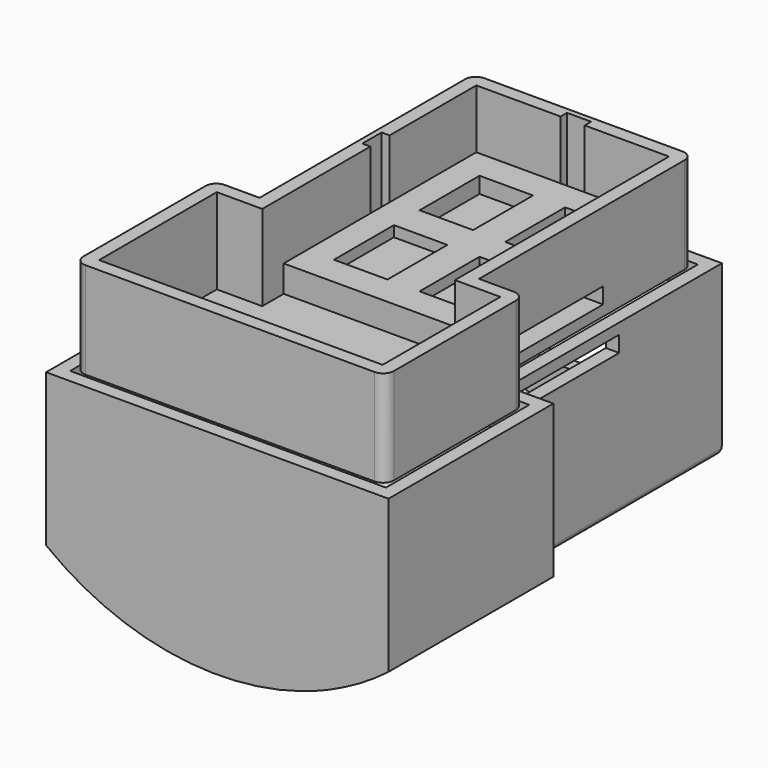
from build123d import *

# Parameters (mm, degrees)
F1_DEPTH  = 2
F2_DEPTH  = 18
F4_DEPTH  = 5
F5_W      = 24
F5_H      = 3
F6_DEPTH  = 41
F7_W      = 10
F7_H      = 14
F8_DEPTH  = 3
F9_DEPTH  = 35
F11_DEPTH = 2
F12_R     = 2
F13_W     = 31
F13_H     = 25
F14_DEPTH = 2.5
F15_R     = 10
F17_DEPTH = 50
F18_DEPTH = 50
F20_DEPTH = 38.5
F21_DEPTH = 38.5
F22_R     = 1
F23_W     = 24
F23_H     = 3
F24_DEPTH = 47
F25_SIZE2 = 20
F25_SIZE  = 2


with BuildPart() as f1:
    # F0 (on Top) → F1 (new body)
    with BuildSketch(Plane.XY):
        Polygon((20.5, -25), (20.5, 25), (-20.5, 25), (-20.5, -25), (-29, -25), (-29, -57.5), (29, -57.5), (29, -25), align=None)
        Polygon((2.25, 22.5), (18, 22.5), (18, -27.5), (26.5, -27.5), (26.5, -55), (-26.5, -55), (-26.5, -27.5), (-18, -27.5), (-18, -2.25), (-19.5, -2.25), (-19.5, 2.25), (-18, 2.25), (-18, 22.5), (-2.25, 22.5), (-2.25, 24), (2.25, 24), align=None, mode=Mode.SUBTRACT)
        Polygon((18, -27.5), (18, 22.5), (2.25, 22.5), (2.25, 24), (-2.25, 24), (-2.25, 22.5), (-18, 22.5), (-18, 2.25), (-19.5, 2.25), (-19.5, -2.25), (-18, -2.25), (-18, -27.5), (-26.5, -27.5), (-26.5, -55), (26.5, -55), (26.5, -27.5), align=None)
    extrude(amount=F1_DEPTH)

    # F0 (on Top) → F2 (join)
    with BuildSketch(Plane.XY):
        Polygon((20.5, -25), (20.5, 25), (-20.5, 25), (-20.5, -25), (-29, -25), (-29, -57.5), (29, -57.5), (29, -25), align=None)
        Polygon((2.25, 22.5), (18, 22.5), (18, -27.5), (26.5, -27.5), (26.5, -55), (-26.5, -55), (-26.5, -27.5), (-18, -27.5), (-18, -2.25), (-19.5, -2.25), (-19.5, 2.25), (-18, 2.25), (-18, 22.5), (-2.25, 22.5), (-2.25, 24), (2.25, 24), align=None, mode=Mode.SUBTRACT)
    extrude(amount=F2_DEPTH)

    # F3 (on face) → F4 (join)
    with BuildSketch(Plane.XY.offset(2)):
        Polygon((18, -22.5), (18, 22.5), (2.25, 22.5), (-2.25, 22.5), (-18, 22.5), (-18, 2.25), (-18, -2.25), (-18, -22.5), align=None)
    extrude(amount=F4_DEPTH)

    # F5 (on face) → F6 (cut, through all)
    with BuildSketch(Plane(origin=(-20.5, 0, 0), x_dir=(0, -1, 0), z_dir=(-1, 0, 0))):
        with Locations((8, 3.5)):
            Rectangle(F5_W, F5_H)
    extrude(amount=-F6_DEPTH, mode=Mode.SUBTRACT)

    # F7 (on face) → F8 (cut)
    with BuildSketch(Plane.XY.offset(7)):
        with Locations((-8, 10)):
            Rectangle(F7_W, F7_H)
        with Locations((8, 10)):
            Rectangle(F7_W, F7_H)
        with Locations((-8, -10)):
            Rectangle(F7_W, F7_H)
        with Locations((8, -10)):
            Rectangle(F7_W, F7_H)
    extrude(amount=-F8_DEPTH, mode=Mode.SUBTRACT)

    # F12
    f12_edges = [f1.edges().sort_by_distance(p)[0] for p in [
        (-29, -57.5, 9),
        (-29, -25, 9),
        (29, -57.5, 9),
        (-20.5, 25, 9),
        (29, -25, 9),
        (20.5, 25, 9),
    ]]
    fillet(f12_edges, radius=F12_R)


with BuildPart() as f9:
    # F0 (on Top) → F9 (new body)
    with BuildSketch(Plane.XY):
        Polygon((-23.5, -22), (-32, -22), (-32, -60.5), (32, -60.5), (32, -22), (23.5, -22), (23.5, 28), (-23.5, 28), align=None)
        with BuildLine():
            Line((-29.5, -58), (-29.5, -24.5))
            Line((-29.5, -24.5), (-23, -24.5))
            ThreePointArc((-23, -24.5), (-21.5857864376, -23.9142135624), (-21, -22.5))
            Line((-21, -22.5), (-21, 25.5))
            Line((-21, 25.5), (21, 25.5))
            Line((21, 25.5), (21, -22.5))
            ThreePointArc((21, -22.5), (21.5857864376, -23.9142135624), (23, -24.5))
            Line((23, -24.5), (29.5, -24.5))
            Line((29.5, -24.5), (29.5, -58))
            Line((29.5, -58), (-29.5, -58))
        make_face(mode=Mode.SUBTRACT)
    extrude(amount=-F9_DEPTH)

    # F10 (on face) → F11 (join)
    with BuildSketch(Plane(origin=(0, 0, -35), x_dir=(1, 0, 0), z_dir=(0, 0, -1))):
        Polygon((32, 60.5), (-32, 60.5), (-32, 22), (-23.5, 22), (-23.5, -28), (23.5, -28), (23.5, 22), (32, 22), align=None)
    extrude(amount=F11_DEPTH)

    # F13 (on face) → F14 (cut, through all)
    with BuildSketch(Plane(origin=(0, 28, 0), x_dir=(-1, 0, 0), z_dir=(0, 1, 0))):
        with Locations((0, -12.5)):
            Rectangle(F13_W, F13_H)
    extrude(amount=-F14_DEPTH, mode=Mode.SUBTRACT)

    # F15
    f15_edges = [f9.edges().sort_by_distance(p)[0] for p in [
        (15.5, 26.75, -25),
        (-15.5, 26.75, -25),
    ]]
    fillet(f15_edges, radius=F15_R)

    # F16 (on face) → F17 (cut, through all)
    with BuildSketch(Plane(origin=(0, 28, 0), x_dir=(-1, 0, 0), z_dir=(0, 1, 0))):
        with BuildLine():
            Line((23.5, -37), (1.547e-07, -37))
            Line((1.547e-07, -37), (-23.5, -37))
            Line((-23.5, -37), (-23.5, -37.7059200294))
            ThreePointArc((-23.5, -37.7059200294), (0, -42.9791666667), (23.5, -37.7059200294))
            Line((23.5, -37.7059200294), (23.5, -37))
        make_face()
        with BuildLine():
            ThreePointArc((1.547e-07, -37), (-12.1269327607, -35.476320292), (-23.5, -31))
            Line((-23.5, -31), (-23.5, -37))
            Line((-23.5, -37), (1.547e-07, -37))
        make_face()
        with BuildLine():
            Line((23.5, -37), (23.5, -31))
            ThreePointArc((23.5, -31), (12.1269329106, -35.4763202538), (1.547e-07, -37))
            Line((1.547e-07, -37), (23.5, -37))
        make_face()
    extrude(amount=-F17_DEPTH, mode=Mode.SUBTRACT)

    # F16 (on face) → F18 (join, through all)
    with BuildSketch(Plane(origin=(0, 28, 0), x_dir=(-1, 0, 0), z_dir=(0, 1, 0))):
        with BuildLine():
            ThreePointArc((23.5, -25), (0, -32.6310333807), (-23.5, -25))
            Line((-23.5, -25), (-23.5, -31))
            ThreePointArc((-23.5, -31), (-12.1269327607, -35.476320292), (1.547e-07, -37))
            ThreePointArc((1.547e-07, -37), (12.1269329106, -35.4763202538), (23.5, -31))
            Line((23.5, -31), (23.5, -25))
        make_face()
    extrude(amount=-F18_DEPTH)

    # F19 (on face) → F20 (cut, through all)
    with BuildSketch(Plane(origin=(0, -22, 0), x_dir=(-1, 0, 0), z_dir=(0, 1, 0))):
        with BuildLine():
            ThreePointArc((-21, -34.9837240518), (-26.6983501126, -32.0711934239), (-32, -28.4869867981))
            Line((-32, -28.4869867981), (-32, -37))
            Line((-32, -37), (-15.5852542827, -37))
            ThreePointArc((-15.5852542827, -37), (-18.3013018384, -36.073511616), (-20.962667627, -35))
            Line((-20.962667627, -35), (-21, -35))
            Line((-21, -35), (-21, -34.9837240518))
        make_face()
        with BuildLine():
            Line((-15.5852542827, -37), (-32, -37))
            Line((-32, -37), (-32, -37.6209894166))
            ThreePointArc((-32, -37.6209894166), (0, -46.8666792548), (32, -37.6209894166))
            Line((32, -37.6209894166), (32, -28.4869867981))
            ThreePointArc((32, -28.4869867981), (9.2454755251, -38.5461837253), (-15.5852542827, -37))
        make_face()
        with BuildLine():
            ThreePointArc((-23.5, -31), (-27.8967129385, -28.3609367759), (-32, -25.2854246794))
            Line((-32, -25.2854246794), (-32, -28.4869867981))
            ThreePointArc((-32, -28.4869867981), (-26.6983501126, -32.0711934239), (-21, -34.9837240518))
            Line((-21, -34.9837240518), (-21, -32.2741110813))
            ThreePointArc((-21, -32.2741110813), (-22.2591181263, -31.6549466933), (-23.5, -31))
        make_face()
        with BuildLine():
            ThreePointArc((32, -25.2854246794), (5.1211905621, -36.6037218611), (-23.5, -31))
            ThreePointArc((-23.5, -31), (-22.2591181263, -31.6549466933), (-21, -32.2741110813))
            Line((-21, -32.2741110813), (-21, -34.9837240518))
            ThreePointArc((-21, -34.9837240518), (-20.9813353917, -34.9918656459), (-20.962667627, -35))
            Line((-20.962667627, -35), (-13.859413167, -35))
            ThreePointArc((-13.859413167, -35), (-7.0014879371, -36.4974237186), (0, -37))
            Line((0, -37), (-15.5852542827, -37))
            ThreePointArc((-15.5852542827, -37), (9.2454755251, -38.5461837253), (32, -28.4869867981))
            Line((32, -28.4869867981), (32, -25.2854246794))
        make_face()
    extrude(amount=-F20_DEPTH, mode=Mode.SUBTRACT)

    # F19 (on face) → F21 (join, through all)
    with BuildSketch(Plane(origin=(0, -22, 0), x_dir=(-1, 0, 0), z_dir=(0, 1, 0))):
        with BuildLine():
            ThreePointArc((-23.5, -31), (-27.8967129385, -28.3609367759), (-32, -25.2854246794))
            Line((-32, -25.2854246794), (-32, -28.4869867981))
            ThreePointArc((-32, -28.4869867981), (-26.6983501126, -32.0711934239), (-21, -34.9837240518))
            Line((-21, -34.9837240518), (-21, -32.2741110813))
            ThreePointArc((-21, -32.2741110813), (-22.2591181263, -31.6549466933), (-23.5, -31))
        make_face()
        with BuildLine():
            Line((-13.859413167, -35), (-20.962667627, -35))
            ThreePointArc((-20.962667627, -35), (-18.3013018384, -36.073511616), (-15.5852542827, -37))
            Line((-15.5852542827, -37), (0, -37))
            ThreePointArc((0, -37), (-7.0014879371, -36.4974237186), (-13.859413167, -35))
        make_face()
        with BuildLine():
            ThreePointArc((32, -25.2854246794), (5.1211905621, -36.6037218611), (-23.5, -31))
            ThreePointArc((-23.5, -31), (-22.2591181263, -31.6549466933), (-21, -32.2741110813))
            Line((-21, -32.2741110813), (-21, -34.9837240518))
            ThreePointArc((-21, -34.9837240518), (-20.9813353917, -34.9918656459), (-20.962667627, -35))
            Line((-20.962667627, -35), (-13.859413167, -35))
            ThreePointArc((-13.859413167, -35), (-7.0014879371, -36.4974237186), (0, -37))
            Line((0, -37), (-15.5852542827, -37))
            ThreePointArc((-15.5852542827, -37), (9.2454755251, -38.5461837253), (32, -28.4869867981))
            Line((32, -28.4869867981), (32, -25.2854246794))
        make_face()
    extrude(amount=-F21_DEPTH)

    # F22
    f22_edges = [f9.edges().sort_by_distance(p)[0] for p in [
        (0, 28, -37),
        (23.5, 3, -31),
        (0, -22, -37),
        (-23.5, 3, -31),
        (-23.5, -22, -15.5),
        (23.5, -22, -15.5),
    ]]
    fillet(f22_edges, radius=F22_R)

    # F23 (on face) → F24 (cut, through all)
    with BuildSketch(Plane.YZ.offset(23.5)):
        with Locations((-8, -3.5)):
            Rectangle(F23_W, F23_H)
    extrude(amount=-F24_DEPTH, mode=Mode.SUBTRACT)

    # F25
    f25_edges = [f9.edges().sort_by_distance(p)[0] for p in [
        (0, -22, -32.631033),
    ]]
    f25_side = f9.faces().sort_by_distance((20.571829, -22, -29.459003))[0]
    chamfer(f25_edges, length=F25_SIZE, length2=F25_SIZE2, reference=f25_side)


solid = Compound([f1.part, f9.part])
